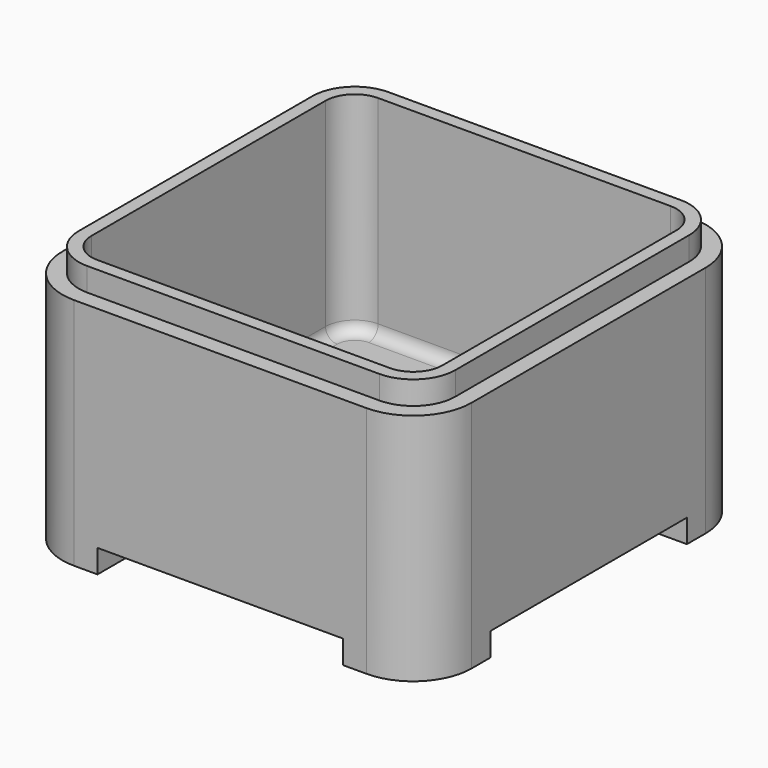
from build123d import *

# Parameters (mm, degrees)
F0_W         = 35
F0_H         = 35
F1_DEPTH     = 11
F2_W         = 21
F2_H         = 7
F2_W_2       = 7
F2_H_2       = 21
F3_DEPTH     = 2
F4_W         = 35
F4_H         = 35
F4_W_2       = 32.2
F4_H_2       = 32.2
F5_DEPTH     = 2
F6_W         = 30
F6_H         = 30
F7_DEPTH     = 18
F8_R         = 1
F9_T1_DEPTH  = 18
F9_T4_ANGLE  = 90
F9_T6_ANGLE  = 90
F9_T8_ANGLE  = 90
F9_T10_ANGLE = 90
F10_R        = 3.6
F11_R        = 5


# Not quite as in the source:
# - a fillet or chamfer that OpenCascade refuses, or shapes differently, is made with other operations: its cross-section is extruded or revolved along the edge and cut away or added


with BuildPart() as f1:
    # F0 (on Top) → F1 (new body, symmetric)
    with BuildSketch(Plane.XY):
        Rectangle(F0_W, F0_H)
    extrude(amount=F1_DEPTH, both=True)

    # F2 (on face) → F3 (cut)
    with BuildSketch(Plane(origin=(0, 0, -11), x_dir=(1, 0, 0), z_dir=(0, 0, -1))):
        with Locations((0, -14)):
            Rectangle(F2_W, F2_H)
        with Locations((-14, 0)):
            Rectangle(F2_W_2, F2_H_2)
        Rectangle(F2_W, F2_H_2)
        with Locations((14, 0)):
            Rectangle(F2_W_2, F2_H_2)
        with Locations((0, 14)):
            Rectangle(F2_W, F2_H)
    extrude(amount=-F3_DEPTH, mode=Mode.SUBTRACT)

    # F4 (on face) → F5 (cut)
    with BuildSketch(Plane.XY.offset(11)):
        Rectangle(F4_W, F4_H)
        Rectangle(F4_W_2, F4_H_2, mode=Mode.SUBTRACT)
    extrude(amount=-F5_DEPTH, mode=Mode.SUBTRACT)

    # F6 (on face) → F7 (cut)
    with BuildSketch(Plane.XY.offset(11)):
        Rectangle(F6_W, F6_H)
    extrude(amount=-F7_DEPTH, mode=Mode.SUBTRACT)

    # F8
    f8_edges = [f1.edges().sort_by_distance(p)[0] for p in [
        (0, 15, -7),
        (-15, 0, -7),
        (0, -15, -7),
        (15, 0, -7),
    ]]
    fillet(f8_edges, radius=F8_R)

    # F9: fillet of radius 2.5 on 4 edges, made by hand

    # F9_s2 → F9_t1 (join)
    with BuildSketch(Plane.XY.offset(-7)):
        with BuildLine():
            ThreePointArc((-12.5, 15), (-14.267766953, 14.267766953), (-15, 12.5))
            Line((-15, 12.5), (-15, 15))
            Line((-15, 15), (-12.5, 15))
        make_face()
        with BuildLine():
            ThreePointArc((15, -12.5), (14.267766953, -14.267766953), (12.5, -15))
            Line((12.5, -15), (15, -15))
            Line((15, -15), (15, -12.5))
        make_face()
        with BuildLine():
            ThreePointArc((15, 12.5), (14.267766953, 14.267766953), (12.5, 15))
            Line((12.5, 15), (15, 15))
            Line((15, 15), (15, 12.5))
        make_face()
        with BuildLine():
            ThreePointArc((-12.5, -15), (-14.267766953, -14.267766953), (-15, -12.5))
            Line((-15, -12.5), (-15, -15))
            Line((-15, -15), (-12.5, -15))
        make_face()
    extrude(amount=F9_T1_DEPTH)

    # F9_s3 → F9_t4 (revolve)
    with BuildSketch(Plane.YZ.offset(-12.5)):
        with BuildLine():
            ThreePointArc((-14, -7), (-14.7071067812, -6.7071067812), (-15, -6))
            Line((-15, -6), (-15, -7))
            Line((-15, -7), (-14, -7))
        make_face()
    revolve(axis=Axis((-12.5, -12.5, -7), (0, 0, -1)), revolution_arc=F9_T4_ANGLE)

    # F9_s5 → F9_t6 (revolve)
    with BuildSketch(Plane.YZ.offset(12.5)):
        with BuildLine():
            ThreePointArc((14, -7), (14.7071067812, -6.7071067812), (15, -6))
            Line((15, -6), (15, -7))
            Line((15, -7), (14, -7))
        make_face()
    revolve(axis=Axis((12.5, 12.5, -7), (0, 0, -1)), revolution_arc=F9_T6_ANGLE)

    # F9_s7 → F9_t8 (revolve)
    with BuildSketch(Plane.XZ.offset(12.5)):
        with BuildLine():
            ThreePointArc((14, -7), (14.7071067812, -6.7071067812), (15, -6))
            Line((15, -6), (15, -7))
            Line((15, -7), (14, -7))
        make_face()
    revolve(axis=Axis((12.5, -12.5, -7), (0, 0, -1)), revolution_arc=F9_T8_ANGLE)

    # F9_s9 → F9_t10 (revolve)
    with BuildSketch(Plane.XZ.offset(-12.5)):
        with BuildLine():
            ThreePointArc((-14, -7), (-14.7071067812, -6.7071067812), (-15, -6))
            Line((-15, -6), (-15, -7))
            Line((-15, -7), (-14, -7))
        make_face()
    revolve(axis=Axis((-12.5, 12.5, -7), (0, 0, -1)), revolution_arc=F9_T10_ANGLE)

    # F10
    f10_edges = [f1.edges().sort_by_distance(p)[0] for p in [
        (-16.1, -16.1, 10),
        (16.1, -16.1, 10),
        (16.1, 16.1, 10),
        (-16.1, 16.1, 10),
    ]]
    fillet(f10_edges, radius=F10_R)

    # F11
    f11_edges = [f1.edges().sort_by_distance(p)[0] for p in [
        (-17.5, -17.5, -1),
        (17.5, -17.5, -1),
        (17.5, 17.5, -1),
        (-17.5, 17.5, -1),
    ]]
    fillet(f11_edges, radius=F11_R)


solid = f1.part
